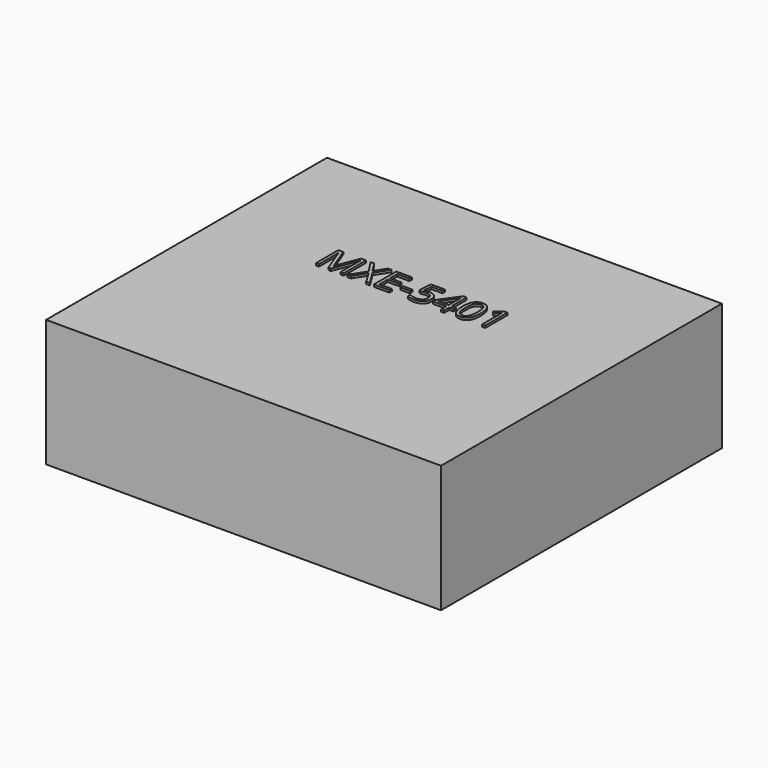
from build123d import *

# Parameters (mm, degrees)
F0_W         = 228.6
F0_H         = 203.2
F1_DEPTH     = 73.66
F2_TEXT_SIZE = 22.6438222594
F3_DEPTH     = 1.27


# Not quite as in the source:
# - Text() gives the source's letters only with a copy of the font that has no kerning and outlines rounded to 1/6400 em; it was checked with that copy


with BuildPart() as f1:
    # F0 (on Top) → F1 (new body)
    with BuildSketch(Plane.XY):
        with Locations((10.7122398913, 35.7262308666)):
            Rectangle(F0_W, F0_H)
    extrude(amount=F1_DEPTH)

    # F2 (on face) → F3 (join)
    with BuildSketch(Plane.XY.offset(73.66)):
        with Locations((-43.7346354875, 51.8284791586)):
            Text('MXE-5401', F2_TEXT_SIZE, font='Open Sans', text_align=(TextAlign.LEFT, TextAlign.BOTTOM))
    extrude(amount=F3_DEPTH)


solid = f1.part
